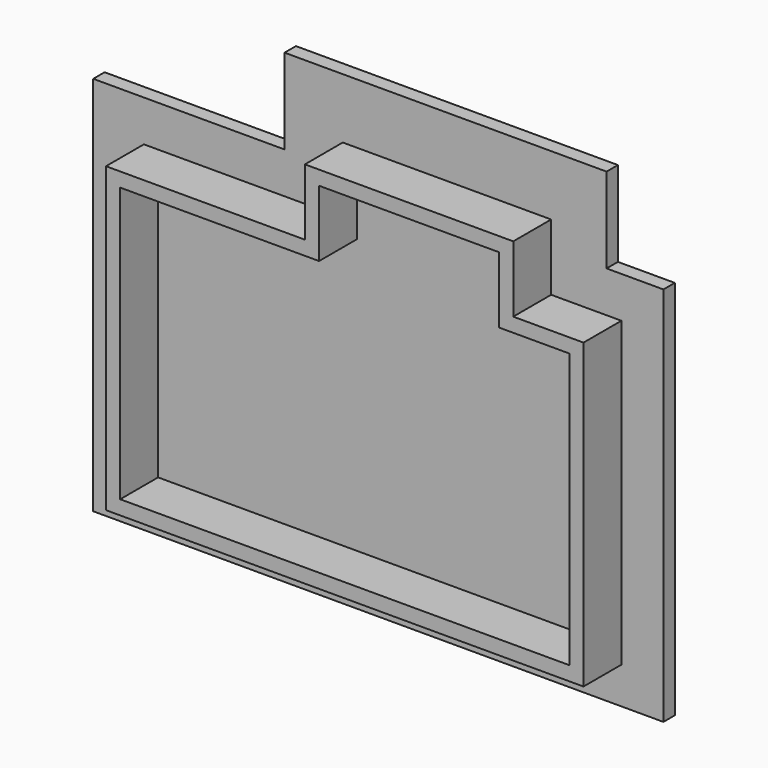
from build123d import *

# Parameters (mm, degrees)
F1_DEPTH     = 1.5
F3_DEPTH     = 5
F4_T         = 1.5
F4_T3_DEPTH  = 4.5
F4_T5_DEPTH  = 10.4166599398
F4_T7_DEPTH  = 10
F4_T9_DEPTH  = 25
F4_T11_DEPTH = 24
F4_T13_DEPTH = 34.9687469041
F4_T15_DEPTH = 53.4166599398
F4_T17_DEPTH = 8


# Not quite as in the source:
# - a shell that OpenCascade refuses in one call is made with other operations: the cavity is built on its own and cut out


with BuildPart() as f1:
    # F0 (on Front) → F1 (new body)
    with BuildSketch(Plane.XZ):
        Polygon((-52.3250011176, 25.3536881179), (-52.3250011176, -14.8463118821), (7.8749988824, -14.8463118821), (7.8749988824, 25.3536881179), (1.8749988824, 25.3536881179), (1.8749988824, 34.3536881179), (-32.1250011176, 34.3536881179), (-32.1250011176, 25.3536881179), align=None)
    extrude(amount=F1_DEPTH)

    # F2 (on face) → F3 (join)
    with BuildSketch(Plane.XZ.offset(1.5)):
        Polygon((-46.9777897949, 21.0005849694), (-46.9777897949, -10.9681619347), (3.4388701449, -10.9681619347), (3.4388701449, 21.0005849694), (-3.9777897949, 21.0005849694), (-3.9777897949, 28.0005849694), (-25.9777897949, 28.0005849694), (-25.9777897949, 21.0005849694), align=None)
    extrude(amount=F3_DEPTH)

    # F4: shell of thickness 1.5, made by hand


with BuildPart() as f4_core1:
    # F4_t2: copy of F1
    add(f1.part)

    # the walls: a layer under each face that stays
    f4_faces = [f4_core1.faces().sort_by_distance(p)[0] for p in [
        (-42.2250011176, -0.75, 25.3536881179),
        (-32.1250011176, -0.75, 29.8536881179),
        (-52.3250011176, -0.75, 5.2536881179),
        (-22.2250011176, 0, 9.7536881179),
        (-2.1583344509, -1.5, 26.1536881179),
        (-15.1250011176, -0.75, 34.3536881179),
        (-22.2250011176, -0.75, -14.8463118821),
        (7.8749988824, -0.75, 5.2536881179),
        (4.8749988824, -0.75, 25.3536881179),
        (1.8749988824, -0.75, 29.8536881179),
        (-0.269459825, -4, 21.0005849694),
        (-3.9777897949, -4, 24.5005849694),
        (-14.9777897949, -4, 28.0005849694),
        (-25.9777897949, -4, 24.5005849694),
        (-36.4777897949, -4, 21.0005849694),
        (-46.9777897949, -4, 5.0162115173),
        (-21.769459825, -4, -10.9681619347),
        (3.4388701449, -4, 5.0162115173),
    ]]
    thicken(f4_faces, amount=-F4_T, mode=Mode.SUBTRACT)

    # F4_s4 → F4_t3 (cut)
    with BuildSketch(Plane.XZ.offset(-1.5)):
        Polygon((-32.1400011176, 25.3686881179), (-32.1250011176, 23.8536881179), (-30.6250011176, 23.8536881179), (-30.6250011176, 25.3536881179), align=None)
        Polygon((1.8899988824, 25.3686881179), (1.8749988824, 23.8536881179), (0.3749988824, 23.8536881179), (0.3749988824, 25.3536881179), align=None)
    extrude(amount=F4_T3_DEPTH, mode=Mode.SUBTRACT)

    # F4_s6 → F4_t5 (cut)
    with BuildSketch(Plane.YZ.offset(-5.4777897949)):
        Polygon((-1.515, 21.0155849694), (0, 21.0005849694), (0, 19.5005849694), (-1.5, 19.5005849694), align=None)
    extrude(amount=F4_T5_DEPTH, mode=Mode.SUBTRACT)

    # F4_s8 → F4_t7 (cut)
    with BuildSketch(Plane.XY.offset(19.5005849694)):
        Polygon((-3.9627897949, -1.515), (-3.9777897949, 0), (-5.4777897949, 0), (-5.4777897949, -1.5), align=None)
        Polygon((-25.9927897949, -1.515), (-25.9777897949, 0), (-24.4777897949, 0), (-24.4777897949, -1.5), align=None)
    extrude(amount=F4_T7_DEPTH, mode=Mode.SUBTRACT)

    # F4_s10 → F4_t9 (cut)
    with BuildSketch(Plane.YZ.offset(-27.4777897949)):
        Polygon((-1.515, 28.0155849694), (0, 28.0005849694), (0, 26.5005849694), (-1.5, 26.5005849694), align=None)
    extrude(amount=F4_T9_DEPTH, mode=Mode.SUBTRACT)

    # F4_s12 → F4_t11 (cut)
    with BuildSketch(Plane.YZ.offset(-48.4777897949)):
        Polygon((-1.515, 21.0155849694), (0, 21.0005849694), (0, 19.5005849694), (-1.5, 19.5005849694), align=None)
    extrude(amount=F4_T11_DEPTH, mode=Mode.SUBTRACT)

    # F4_s14 → F4_t13 (cut)
    with BuildSketch(Plane.XY.offset(-12.4681619347)):
        Polygon((-46.9927897949, -1.515), (-46.9777897949, 0), (-45.4777897949, 0), (-45.4777897949, -1.5), align=None)
        Polygon((3.4538701449, -1.515), (3.4388701449, 0), (1.9388701449, 0), (1.9388701449, -1.5), align=None)
    extrude(amount=F4_T13_DEPTH, mode=Mode.SUBTRACT)

    # F4_s16 → F4_t15 (cut)
    with BuildSketch(Plane.YZ.offset(-48.4777897949)):
        Polygon((-1.515, -10.9831619347), (0, -10.9681619347), (0, -9.4681619347), (-1.5, -9.4681619347), align=None)
    extrude(amount=F4_T15_DEPTH, mode=Mode.SUBTRACT)

    # F4_s18 → F4_t17 (cut)
    with BuildSketch(Plane.XZ):
        Polygon((-3.9627897949, 21.0155849694), (-3.9777897949, 19.5005849694), (-5.4777897949, 19.5005849694), (-5.4777897949, 21.0005849694), align=None)
        Polygon((-25.9927897949, 21.0155849694), (-24.4777897949, 21.0005849694), (-24.4777897949, 19.5005849694), (-25.9777897949, 19.5005849694), align=None)
    extrude(amount=F4_T17_DEPTH, mode=Mode.SUBTRACT)


with BuildPart() as f1_1:
    add(f1.part)

    # what is left inside the walls is the cavity
    f4_cavity = [f4_core1.part.solids().sort_by_distance(p)[0] for p in [
        (-21.76946, -1.515, 2.52142),
    ]]
    add(f4_cavity, mode=Mode.SUBTRACT)


solid = f1_1.part
